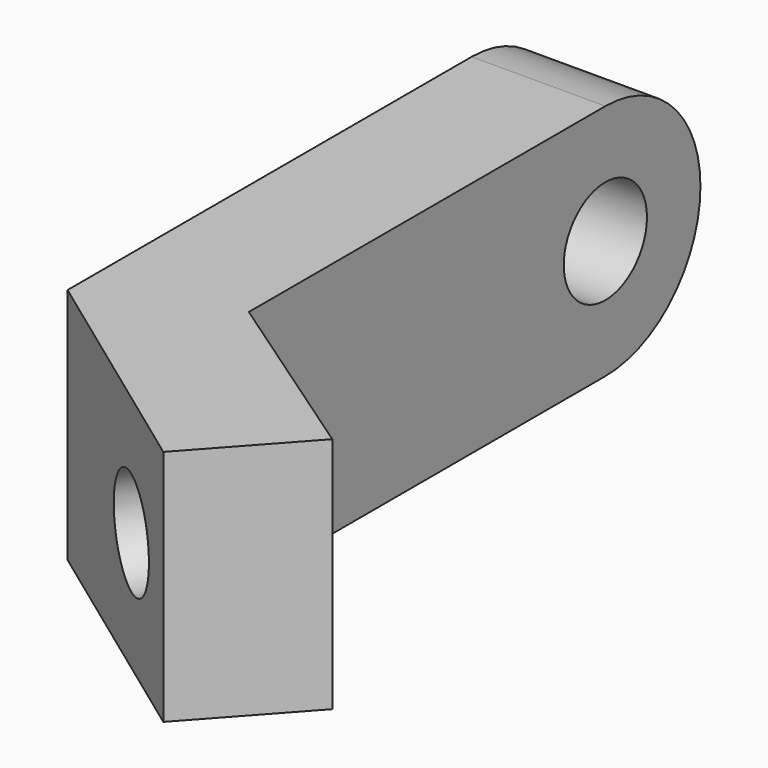
from build123d import *

# Parameters (mm, degrees)
F1_DEPTH = 8
F2_R     = 3.99999
F3_R     = 1.75
F4_DEPTH = 4.5
F5_R     = 1.75
F6_DEPTH = 4.84


# Not quite as in the source:
# - a fillet or chamfer is up to 0.001 mm smaller than in the source, because OpenCascade refuses the exact size
# - a feature names something its author has since deleted; it is built from what else it names


with BuildPart() as f1:
    # F0 (on Top) → F1 (new body)
    with BuildSketch(Plane.XY):
        Polygon((4.5, 0), (0, 0), (0, -21), (7.7216494845, -26.6237113402), (10.7371134021, -23.2835051546), (4.5, -19), align=None)
    extrude(amount=F1_DEPTH)

    # F2 (radius 4 in the source; OpenCascade refuses exactly that, so slightly less here)
    f2_edges = [f1.edges().sort_by_distance(p)[0] for p in [
        (2.25, 0, 8),
        (2.25, 0, 0),
    ]]
    fillet(f2_edges, radius=F2_R)

    # F3 (on face) → F4 (cut)
    with BuildSketch(Plane.YZ.offset(4.5)):
        with Locations((-4, 4)):
            Circle(F3_R)
    extrude(amount=-F4_DEPTH, mode=Mode.SUBTRACT)

    # F5 (on face) → F6 (cut)
    with BuildSketch(Plane(origin=(-7.4244465835, -10.8105660241, 0), x_dir=(-0.8243201098, 0.5661239763, 0), z_dir=(0.5661239763, 0.8243201098, 0))):
        with Locations((-18.248982531, 4)):
            Circle(F5_R)
    extrude(amount=-F6_DEPTH, mode=Mode.SUBTRACT)


solid = f1.part
